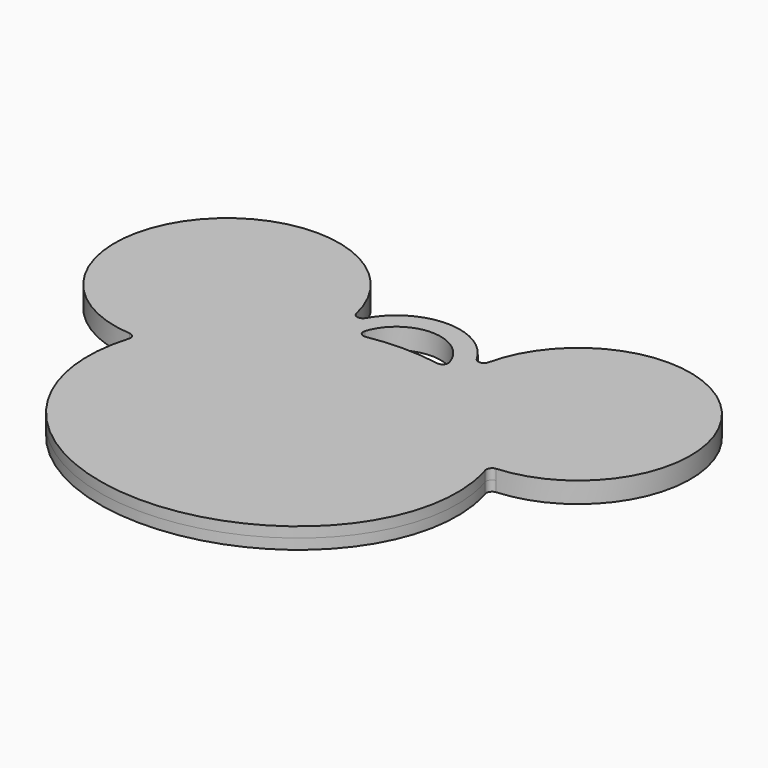
from build123d import *

# Parameters (mm, degrees)
F1_DEPTH      = 1.3716
F3_DEPTH      = 1.3716
F3_DEPTH_BACK = 1.3716
F4_R          = 0.762


# Not quite as in the source:
# - a feature names something its author has since deleted; it is built from what else it names


with BuildPart() as f1:
    # F0 (on Top) → F1 (new body, symmetric)
    with BuildSketch(Plane.XY):
        with BuildLine():
            ThreePointArc((-8.4232286975, 20.3914902339), (-33.3355583029, 32.417888511), (-23.260879727, 6.6543624814))
            add(Edge.make_bspline(
                [(-23.260879727, 6.6543624814), (-33.5330229603, -21.7229145667), (0, -21.7229145667), (33.5330229603, -21.7229145667), (23.260879727, 6.6543624814)],
                knots=[2.8302582369, 2.8302582369, 2.8302582369, 4.7123889804, 4.7123889804, 6.5945197238, 6.5945197238, 6.5945197238], degree=2, weights=[1, 0.5889273409, 1, 0.5889273409, 1]))
            ThreePointArc((23.260879727, 6.6543624814), (33.3355583029, 32.417888511), (8.4232286975, 20.3914902339))
            add(Edge.make_bspline(
                [(8.4232286975, 20.3914902339), (0, 23.1412717688), (-8.4232286975, 20.3914902339)],
                knots=[1.2188651396, 1.2188651396, 1.2188651396, 1.922727514, 1.922727514, 1.922727514], degree=2, weights=[1, 0.9387087617, 1]))
        make_face()
    extrude(amount=F1_DEPTH, both=True)

    # F2 (on Top) → F3 (join, two sides)
    with BuildSketch(Plane.XY) as f3_sk:
        with BuildLine():
            add(Edge.make_bspline(
                [(8.4232286975, 20.3914902339), (7.1587937107, 20.8042678164), (5.8509839512, 21.0909933818)],
                knots=[1.2188651396, 1.2188651396, 1.2188651396, 1.3290021299, 1.3290021299, 1.3290021299], degree=2, weights=[1, 0.9984841136, 1]))
            ThreePointArc((8.4232286975, 20.3914902339), (0, 28.8958069319), (-8.4232286975, 20.3914902339))
            add(Edge.make_bspline(
                [(-5.8509839512, 21.0909933818), (-7.1587937107, 20.8042678164), (-8.4232286975, 20.3914902339)],
                knots=[1.8125905237, 1.8125905237, 1.8125905237, 1.922727514, 1.922727514, 1.922727514], degree=2, weights=[1, 0.9984841136, 1]))
            ThreePointArc((-5.8509839512, 21.0909933818), (0, 26.3558069319), (5.8509839512, 21.0909933818))
        make_face()
    extrude(amount=F3_DEPTH)
    extrude(f3_sk.sketch, amount=-F3_DEPTH_BACK)

    # F4
    f4_edges = [f1.edges().sort_by_distance(p)[0] for p in [
        (5.850984, 21.090993, -0.6858),
        (-5.850984, 21.090993, -0.6858),
        (23.26088, 6.654362, 0.6858),
        (23.26088, 6.654362, -0.6858),
        (-23.26088, 6.654362, 0.6858),
        (-23.26088, 6.654362, -0.6858),
        (8.382226, 21.306212, 0),
        (-8.382226, 21.306212, 0),
        (-5.850984, 21.090993, 0.6858),
        (5.850984, 21.090993, 0.6858),
    ]]
    fillet(f4_edges, radius=F4_R)


solid = f1.part
